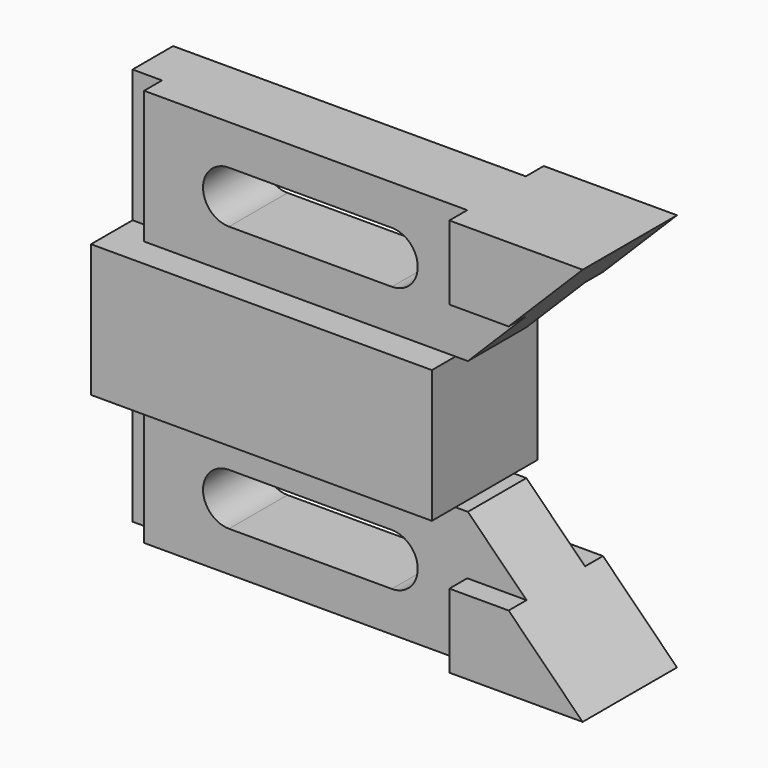
from build123d import *

# Parameters (mm, degrees)
F1_DEPTH = 104.648
F2_W     = 75.946
F2_H     = 4.826
F2_W_2   = 6.35
F3_DEPTH = 28.575
F5_DEPTH = 22.099
F7_DEPTH = 26.925
F9_DEPTH = 28.449


# Not quite as in the source:
# - a pattern or mirror of a feature is missing from the dataset's text; its kind, count and spacing are read off the source's solid


with BuildPart() as f1:
    # F0 (on Right) → F1 (new body)
    with BuildSketch(Plane.YZ):
        Polygon((7.874, -14.2875), (14.224, -14.2875), (14.224, 14.2875), (7.874, 14.2875), (-7.874, 14.2875), (-14.224, 14.2875), (-14.224, -14.2875), (-7.874, -14.2875), align=None)
        Polygon((-7.874, 14.2875), (7.874, 14.2875), (7.874, 26.924), (12.7, 26.924), (12.7, 42.8625), (0, 42.8625), (-12.7, 42.8625), (-12.7, 26.924), (-7.874, 26.924), align=None)
        Polygon((7.874, -26.924), (7.874, -14.2875), (-7.874, -14.2875), (-7.874, -26.924), (-12.7, -26.924), (-12.7, -42.8625), (0, -42.8625), (12.7, -42.8625), (12.7, -26.924), align=None)
    extrude(amount=-F1_DEPTH)

    # F2 (on face) → F3 (cut)
    with BuildSketch(Plane.XY.offset(42.8625)):
        Polygon((-98.298, -7.874), (-104.648, -7.874), (-104.648, -12.7), (-28.702, -12.7), (-28.702, -7.874), align=None)
        with Locations((-66.675, 10.287)):
            Rectangle(F2_W, F2_H)
        with Locations((-101.473, -5.461)):
            Rectangle(F2_W_2, F2_H)
    f3 = extrude(amount=-F3_DEPTH, mode=Mode.SUBTRACT)

    # F3_copies: F3 across plane
    add(f3.mirror(Plane(origin=(0, 0, 0), x_dir=(-1, 0, 0), z_dir=(0, 0, -1))), mode=Mode.SUBTRACT)

    # F4 (on face) → F5 (cut, through all)
    with BuildSketch(Plane.XZ.offset(7.874)):
        with BuildLine():
            ThreePointArc((-80.01, -34.2265), (-76.0586873067, -32.5898126933), (-74.422, -28.6385))
            ThreePointArc((-74.422, -28.6385), (-76.0586873067, -24.6871873067), (-80.01, -23.0505))
            ThreePointArc((-80.01, -23.0505), (-85.598, -28.6385), (-80.01, -34.2265))
        make_face()
        with BuildLine():
            ThreePointArc((-80.01, -23.0505), (-76.0586873067, -24.6871873067), (-74.422, -28.6385))
            ThreePointArc((-74.422, -28.6385), (-76.0586873067, -32.5898126933), (-80.01, -34.2265))
            Line((-80.01, -34.2265), (-44.958, -34.2265))
            ThreePointArc((-44.958, -34.2265), (-50.546, -28.6385), (-44.958, -23.0505))
            Line((-44.958, -23.0505), (-80.01, -23.0505))
        make_face()
        with BuildLine():
            ThreePointArc((-39.37, -28.6385), (-41.0066873067, -24.6871873067), (-44.958, -23.0505))
            ThreePointArc((-44.958, -23.0505), (-50.546, -28.6385), (-44.958, -34.2265))
            ThreePointArc((-44.958, -34.2265), (-41.0066873067, -32.5898126933), (-39.37, -28.6385))
        make_face()
    f5 = extrude(amount=-F5_DEPTH, mode=Mode.SUBTRACT)

    # F5_copies: F5 across plane
    add(f5.mirror(Plane.XY), mode=Mode.SUBTRACT)

    # F6 (on face) → F7 (cut, through all)
    with BuildSketch(Plane.XZ.offset(12.7)):
        Polygon((0, -14.2875), (-28.575, -14.2875), (0, -42.8625), align=None)
    f7 = extrude(amount=-F7_DEPTH, mode=Mode.SUBTRACT)

    # F7_copies: F7 across plane
    add(f7.mirror(Plane.XY), mode=Mode.SUBTRACT)

    # F8 (on face) → F9 (cut, through all)
    with BuildSketch(Plane.XZ.offset(14.224)):
        Polygon((-31.242, 14.2875), (-31.242, 0), (-31.242, -14.2875), (0, -14.2875), (0, 14.2875), align=None)
    extrude(amount=-F9_DEPTH, mode=Mode.SUBTRACT)


solid = f1.part
